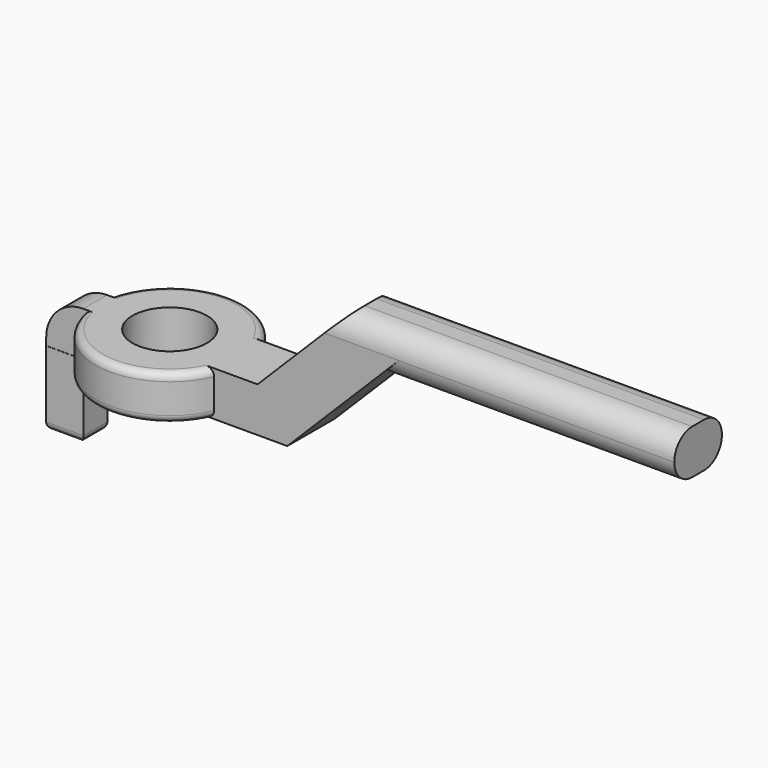
from build123d import *

# Parameters (mm, degrees)
F1_R     = 5
F2_DEPTH = 6
F4_DEPTH = 10
F5_R     = 5
F6_W     = 10
F6_H     = 8
F7_DEPTH = 6
F9_DEPTH = 6
F10_SIZE = 5.99999
F11_R    = 2.99999
F12_R    = 1
F13_R    = 1


# Not quite as in the source:
# - a fillet or chamfer is up to 0.001 mm smaller than in the source, because OpenCascade refuses the exact size


with BuildPart() as f2:
    # F1 (on offset) → F2 (new body)
    with BuildSketch(Plane.XY.offset(27)):
        with BuildLine():
            ThreePointArc((9.1651513899, -4), (9.7890631293, -2.0430964369), (10, 0))
            ThreePointArc((10, 0), (9.7890631293, 2.0430964369), (9.1651513899, 4))
            ThreePointArc((9.1651513899, 4), (-1.048861935, 9.9448423135), (-9.7979589711, 2))
            ThreePointArc((-9.7979589711, 2), (-9.9493615301, 1.0050896201), (-10, 0))
            ThreePointArc((-10, 0), (-9.9493615301, -1.0050896201), (-9.7979589711, -2))
            ThreePointArc((-9.7979589711, -2), (-1.048861935, -9.9448423135), (9.1651513899, -4))
        make_face()
        Circle(F1_R, mode=Mode.SUBTRACT)
        with BuildLine():
            Line((25, 0), (10, 0))
            ThreePointArc((10, 0), (9.7890631293, -2.0430964369), (9.1651513899, -4))
            Line((9.1651513899, -4), (25, -4))
            Line((25, -4), (25, 0))
        make_face()
        with BuildLine():
            ThreePointArc((9.1651513899, 4), (9.7890631293, 2.0430964369), (10, 0))
            Line((10, 0), (25, 0))
            Line((25, 0), (25, 4))
            Line((25, 4), (9.1651513899, 4))
        make_face()
        with BuildLine():
            ThreePointArc((-10, 0), (-9.9493615301, 1.0050896201), (-9.7979589711, 2))
            Line((-9.7979589711, 2), (-15, 2))
            Line((-15, 2), (-15, 0))
            Line((-15, 0), (-10, 0))
        make_face()
        with BuildLine():
            Line((-15, -2), (-9.7979589711, -2))
            ThreePointArc((-9.7979589711, -2), (-9.9493615301, -1.0050896201), (-10, 0))
            Line((-10, 0), (-15, 0))
            Line((-15, 0), (-15, -2))
        make_face()
    extrude(amount=F2_DEPTH)

    # F3 (on offset) → F4 (join)
    with BuildSketch(Plane.XY.offset(27)):
        Polygon((-10, -2.0203573131), (-10, 2.0309494015), (-15, 1.9722348321), (-15, -2.0203573131), align=None)
    extrude(amount=-F4_DEPTH)

    # F5
    f5_edges = [f2.edges().sort_by_distance(p)[0] for p in [
        (-15, 0, 33),
    ]]
    fillet(f5_edges, radius=F5_R)

    # F6 (on face) → F7 (join)
    with BuildSketch(Plane.XY.offset(33)):
        with Locations((20, 0)):
            Rectangle(F6_W, F6_H)
    extrude(amount=F7_DEPTH)

    # F8 (on face) → F9 (join)
    with BuildSketch(Plane.XY.offset(39)):
        Polygon((21, 4), (21, 0), (21, -4), (71, -4), (71, 4), align=None)
    extrude(amount=F9_DEPTH)

    # F10 (size 6 in the source; OpenCascade refuses exactly that, so slightly less here)
    f10_edges = [f2.edges().sort_by_distance(p)[0] for p in [
        (25, 0, 27),
        (15, 0, 39),
        (21, 0, 45),
        (25, 0, 39),
    ]]
    chamfer(f10_edges, length=F10_SIZE)

    # F11 (radius 3 in the source; OpenCascade refuses exactly that, so slightly less here)
    f11_edges = [f2.edges().sort_by_distance(p)[0] for p in [
        (48.999995, -4, 45),
        (50.999995, -4, 39),
        (50.999995, 4, 39),
        (48.999995, 4, 45),
    ]]
    fillet(f11_edges, radius=F11_R)

    # F12
    f12_edges = [f2.edges().sort_by_distance(p)[0] for p in [
        (-1.048862, -9.944842, 33),
        (-1.048862, -9.944842, 27),
        (-1.048862, 9.944842, 33),
        (-1.048862, 9.944842, 27),
    ]]
    fillet(f12_edges, radius=F12_R)

    # F13
    f13_edges = [f2.edges().sort_by_distance(p)[0] for p in [
        (-12.5, -2.020357, 17),
        (-15, -0.024061, 17),
        (-12.5, 2.001592, 17),
        (-10, 0.005296, 17),
    ]]
    fillet(f13_edges, radius=F13_R)


solid = f2.part
